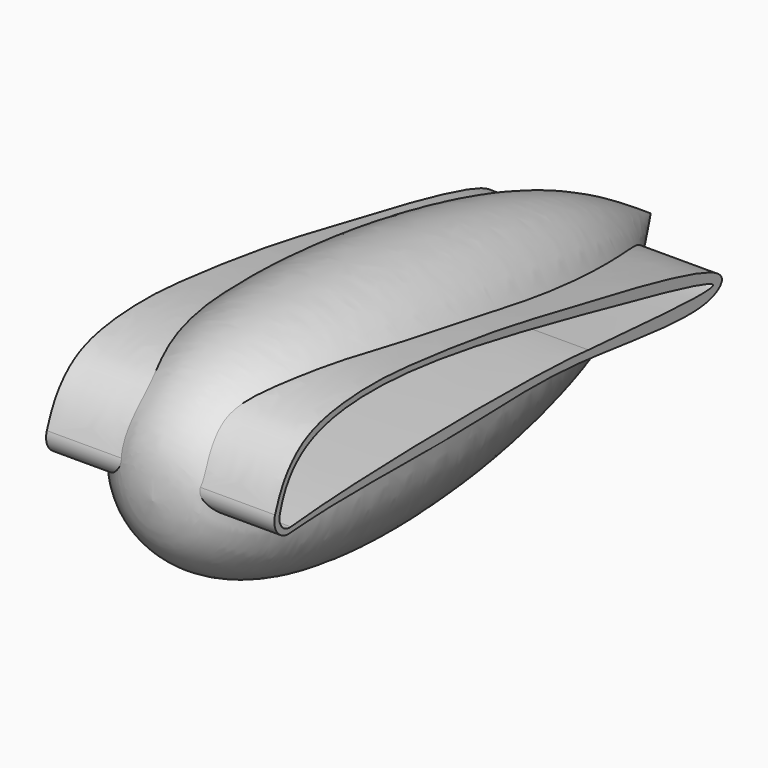
from build123d import *

# Parameters (mm, degrees)
F5_DEPTH = 111.76
F6_DEPTH = 326.136


with BuildPart() as f1:
    # F0 (on Right) → F1 (revolve)
    with BuildSketch(Plane.YZ):
        with BuildLine():
            add(Edge.make_bspline(
                [(0, 0), (1.2629827023, 14.9905999022), (4.4503594239, 52.8222258515), (103.5524753502, 131.2753056375), (468.0764268076, 95.3144986391), (568.5368175296, 27.6555810555), (609.6, 0)],
                knots=[0, 0, 0, 0, 0.1384169551, 0.3493214752, 0.7340351675, 1, 1, 1, 1], degree=3))
            Line((0, 0), (609.6, 0))
        make_face()
    revolve(axis=Axis((0, 304.8, 0), (0, 1, 0)))

    # F3 (on Right) → F5 (join, symmetric)
    with BuildSketch(Plane.YZ):
        with BuildLine():
            add(Edge.make_bspline(
                [(10.0180897862, 20.0675204396), (12.9036061679, 28.0863992709), (18.9567463951, 44.9081363912), (40.8411580479, 69.8428959764), (75.5390116217, 81.846118244), (125.0629221536, 85.3065250037), (173.6523105789, 82.8085327515), (280.9237290105, 69.8862606709), (364.6680467655, 52.844203247), (538.6085038972, 20.5318460332), (562.9209204198, -0.1964214501), (530.8916963429, -22.7306704833), (366.3804462694, 7.6238258667), (247.0910750943, -2.4066068043), (96.8269195046, 1.6135643432), (46.5008001014, -1.7804422991), (25.9270556271, -3.1679410022)],
                knots=[0, 0, 0, 0, 0.0432596649, 0.0907486852, 0.1416764608, 0.2002183109, 0.2603165439, 0.3455748941, 0.43081491, 0.5424172154, 0.5798451579, 0.6210524899, 0.7285736745, 0.8273625774, 0.9294243573, 1, 1, 1, 1], degree=3))
            ThreePointArc((10.0180897862, 20.0675204396), (12.1765524111, 4.4813430784), (25.9270556271, -3.1679410022))
        make_face()
    extrude(amount=F5_DEPTH, both=True)

    # F4 (on offset) → F6 (cut, symmetric)
    with BuildSketch(Plane.YZ.offset(111.76)):
        with BuildLine():
            add(Edge.make_bspline(
                [(15.7258266677, 17.6259054527), (25.1218080226, 55.3636780478), (100.2303747073, 100.0439387405), (368.7005055306, 43.7489926546), (621.221483251, -10.8903573898), (468.9769449321, 0.9076995702), (393.7, 6.35)],
                knots=[0.0246233793, 0.0246233793, 0.0246233793, 0.0246233793, 0.1966407732, 0.5286341469, 0.7660519635, 1, 1, 1, 1], degree=3))
            ThreePointArc((15.7258266677, 17.6259054527), (17.7717954355, 7.0971625816), (27.1484189149, 1.8895386733))
            ThreePointArc((27.1484189149, 1.8895386733), (28.247943523, 1.859074932), (29.3459801953, 1.9238659012))
            add(Edge.make_bspline(
                [(393.7, 6.35), (345.9854504861, 12.361468203), (134.1860087973, 12.6819515476), (29.3459801953, 1.9238659012)],
                knots=[0, 0, 0, 0, 360.7381833424, 360.7381833424, 360.7381833424, 360.7381833424], degree=3))
        make_face()
    extrude(amount=F6_DEPTH, both=True, mode=Mode.SUBTRACT)


solid = f1.part
